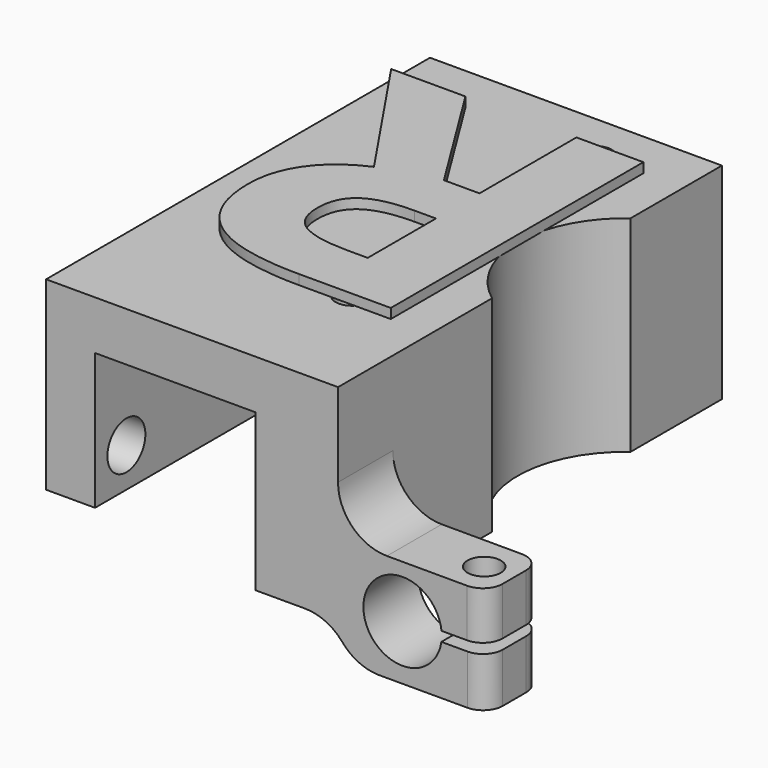
from build123d import *

# Parameters (mm, degrees)
F1_DEPTH      = 7
F2_DEPTH      = 42
F3_R          = 1.7
F3_R_2        = 11
F4_DEPTH      = 21.001
F5_R          = 4
F6_DEPTH      = 10
F7_DEPTH      = 21.001
F8_R          = 1.4
F9_DEPTH      = 11.0273629037
F8_R_2        = 1.7
F10_DEPTH     = 4.9110969969
F11_R         = 5
F12_R         = 5
F13_R         = 5
F14_R         = 2
F15_R         = 2.2
F15_R_2       = 2.4255023423
F16_DEPTH     = 6
F17_TEXT_SIZE = 45.156212112
F18_DEPTH     = 1


# Not quite as in the source:
# - a feature names something its author has since deleted; it is built from what else it names
# - Text() gives the source's letters only with a copy of the font that has no kerning and outlines rounded to 1/6400 em; it was checked with that copy


with BuildPart() as f1:
    # F0 (on Front) → F1 (new body)
    with BuildSketch(Plane.XZ):
        Polygon((-18.6721007523, 29.8099789735), (-18.6721007523, 10.8925135386), (-13.6721007523, 10.8925135386), (-13.6721007523, 24.8099789735), (2.7278992477, 24.8099789735), (2.7278992477, 8.8099789735), (11.1380548998, 8.8099789735), (11.1380548998, 16.2656020473), (11.1380548998, 29.8099789735), align=None)
        Polygon((26.3263195603, 16.2417280634), (11.1380548998, 16.2656020473), (11.1380548998, 8.8099789735), (12.5533044869, 5.2860832236), (26.3553367778, 5.2860832236), (26.3553367778, 10.343908232), (19.6860510706, 10.343908232), (19.6860510706, 11.3388913612), (26.3263195603, 11.3388913612), align=None)
    extrude(amount=F1_DEPTH)

    # F0 (on Front) → F2 (join)
    with BuildSketch(Plane.XZ):
        Polygon((-18.6721007523, 29.8099789735), (-18.6721007523, 10.8925135386), (-13.6721007523, 10.8925135386), (-13.6721007523, 24.8099789735), (2.7278992477, 24.8099789735), (2.7278992477, 8.8099789735), (11.1380548998, 8.8099789735), (11.1380548998, 16.2656020473), (11.1380548998, 29.8099789735), align=None)
    extrude(amount=-F2_DEPTH)

    # F3 (on face) → F4 (cut, through all)
    with BuildSketch(Plane(origin=(0, 0, 8.8099789735), x_dir=(1, 0, 0), z_dir=(0, 0, -1))):
        with Locations((2.1850741468, -6)):
            Circle(F3_R)
        with Locations((2.1850741468, -37)):
            Circle(F3_R)
        with Locations((17.6850741468, -21.5)):
            Circle(F3_R_2)
    extrude(amount=-F4_DEPTH, mode=Mode.SUBTRACT)

    # F5 (on face) → F6 (cut)
    with BuildSketch(Plane.XZ.offset(7)):
        with Locations((17.7278992477, 10.8989789735)):
            Circle(F5_R)
    extrude(amount=-F6_DEPTH, mode=Mode.SUBTRACT)

    # F3 (on face) → F7 (cut, through all)
    with BuildSketch(Plane(origin=(0, 0, 8.8099789735), x_dir=(1, 0, 0), z_dir=(0, 0, -1))):
        with Locations((2.1850741468, -6)):
            Circle(F3_R)
        with Locations((2.1850741468, -37)):
            Circle(F3_R)
        with Locations((17.6850741468, -21.5)):
            Circle(F3_R_2)
    extrude(amount=-F7_DEPTH, mode=Mode.SUBTRACT)

    # F8 (on face) → F9 (cut, through all)
    with BuildSketch(Plane(origin=(0.0255948751, 0, 16.2830693945), x_dir=(0.9999987646, 0, -0.0015718685), z_dir=(0.0015718685, 0, 0.9999987646))):
        with Locations((23.3007571768, -3.5767070949)):
            Circle(F8_R)
    extrude(amount=-F9_DEPTH, mode=Mode.SUBTRACT)

    # F8 (on face) → F10 (cut, through all)
    with BuildSketch(Plane(origin=(0.0255948751, 0, 16.2830693945), x_dir=(0.9999987646, 0, -0.0015718685), z_dir=(0.0015718685, 0, 0.9999987646))):
        with Locations((23.3007571768, -3.5767070949)):
            Circle(F8_R_2)
        with Locations((23.3007571768, -3.5767070949)):
            Circle(F8_R, mode=Mode.SUBTRACT)
    extrude(amount=-F10_DEPTH, mode=Mode.SUBTRACT)

    # F11
    f11_edges = [f1.edges().sort_by_distance(p)[0] for p in [
        (11.138055, -3.5, 16.265602),
    ]]
    fillet(f11_edges, radius=F11_R)

    # F12
    f12_edges = [f1.edges().sort_by_distance(p)[0] for p in [
        (11.138055, -3.5, 8.809979),
    ]]
    fillet(f12_edges, radius=F12_R)

    # F13
    f13_edges = [f1.edges().sort_by_distance(p)[0] for p in [
        (12.553304, -3.5, 5.286083),
    ]]
    fillet(f13_edges, radius=F13_R)

    # F14
    f14_edges = [f1.edges().sort_by_distance(p)[0] for p in [
        (26.32632, -7, 13.79031),
        (26.355337, -7, 7.814996),
        (26.32632, 0, 13.79031),
        (26.355337, 0, 7.814996),
    ]]
    fillet(f14_edges, radius=F14_R)

    # F15 (on face) → F16 (cut)
    with BuildSketch(Plane(origin=(-18.6721007523, 0, 0), x_dir=(0, -1, 0), z_dir=(-1, 0, 0))):
        with Locations((-38, 14.8925135386)):
            Circle(F15_R)
        with Locations((3, 14.8925135386)):
            Circle(F15_R_2)
    extrude(amount=-F16_DEPTH, mode=Mode.SUBTRACT)

    # F17 (on face) → F18 (join)
    with BuildSketch(Plane.XY.offset(29.8099789735)):
        with Locations(Location((11.1380548998, 37.0447599313), (0, 0, 180))):
            Text('R', F17_TEXT_SIZE, font='Open Sans', font_style=FontStyle.BOLD, text_align=(TextAlign.LEFT, TextAlign.BOTTOM))
    extrude(amount=F18_DEPTH)


solid = f1.part
